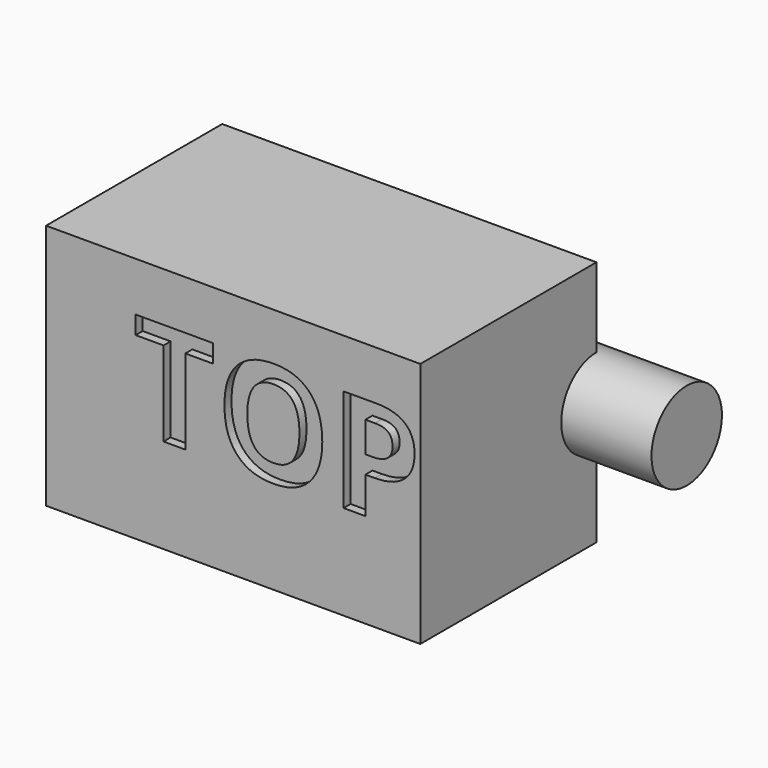
from build123d import *

# Parameters (mm, degrees)
F0_W         = 63
F0_H         = 10
F2_W         = 85
F2_H         = 56
F3_DEPTH     = 50
F4_TEXT_SIZE = 32.688075185
F5_DEPTH     = 2


# Not quite as in the source:
# - Text() gives the source's letters only with a copy of the font that has no kerning and outlines rounded to 1/6400 em; it was checked with that copy


with BuildPart() as f1:
    # F0 (on Front) → F1 (revolve)
    with BuildSketch(Plane.XZ):
        with Locations((31.5, 5)):
            Rectangle(F0_W, F0_H)
    revolve(axis=Axis((31.5, 0, 0), (1, 0, 0)))


with BuildPart() as f3:
    # F2 (on Front) → F3 (new body)
    with BuildSketch(Plane.XZ):
        Rectangle(F2_W, F2_H)
    extrude(amount=F3_DEPTH)

    # F4 (on face) → F5 (cut)
    with BuildSketch(Plane.XZ.offset(50)):
        with Locations((-22.816600278, -6.4869453199)):
            Text('TOP', F4_TEXT_SIZE, font='Open Sans', font_style=FontStyle.BOLD, text_align=(TextAlign.LEFT, TextAlign.BOTTOM))
    extrude(amount=-F5_DEPTH, mode=Mode.SUBTRACT)


solid = Compound([f1.part, f3.part])
